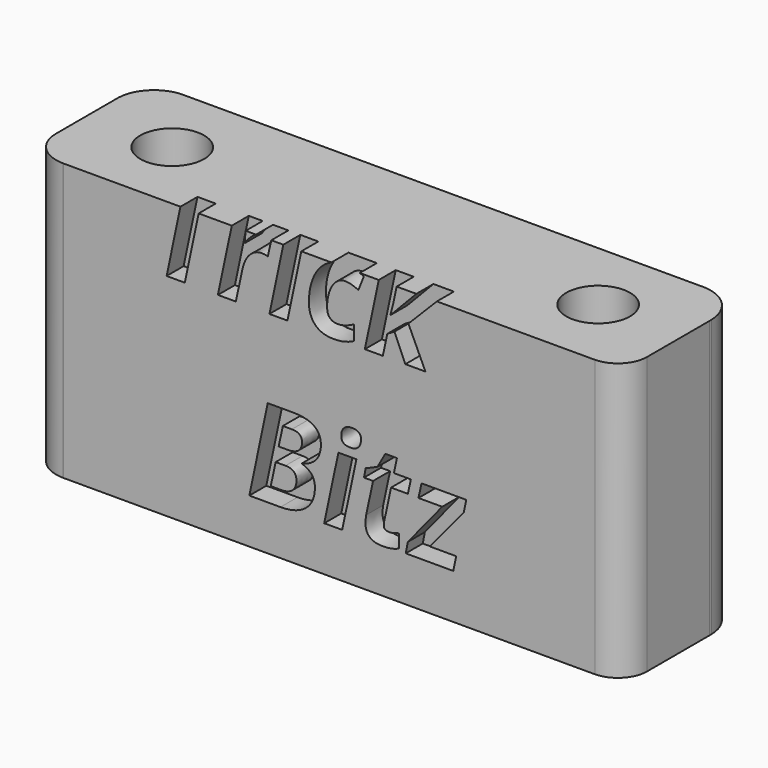
from build123d import *

# Parameters (mm, degrees)
F1_DEPTH     = 13
F2_R         = 1.375
F3_DEPTH     = 10
F4_R         = 1.5
F5_DEPTH     = 10
F6_DEPTH     = 2
F7_TEXT_SIZE = 5.7462564049
F8_DEPTH     = 1
F9_DEPTH     = 2


# Not quite as in the source:
# - Text() gives the source's letters only with a copy of the font that has no kerning and outlines rounded to 1/6400 em; it was checked with that copy


with BuildPart() as f1:
    # F0 (on Top) → F1 (new body)
    with BuildSketch(Plane.XY):
        with BuildLine():
            ThreePointArc((-28, 1.6615508357), (-27.5071954744, 0.4933001093), (-26.3391539245, 0))
            Line((-26.3391539245, 0), (-26.2933354825, 0))
            Line((-26.2933354825, 0), (-1.3435167493, 0))
            ThreePointArc((-1.3435167493, 0), (-0.3933494407, 0.4100272729), (0, 1.3672192581))
            Line((0, 1.3672192581), (0, 5.037621595))
            Line((0, 5.037621595), (0, 5.1521943092))
            ThreePointArc((0, 5.1521943092), (-0.5268150374, 6.4133231242), (-1.7612340162, 7))
            Line((-1.7612340162, 7), (-26.2933354825, 7))
            ThreePointArc((-26.2933354825, 7), (-27.4858583006, 6.507821672), (-28, 5.3246021271))
            Line((-28, 5.3246021271), (-28, 1.6615508357))
        make_face()
        with BuildLine():
            Line((-26.2933354825, 0), (-26.3391539245, 0))
            ThreePointArc((-26.3391539245, 0), (-26.3162447035, -0.0001558454), (-26.2933354825, 0))
        make_face()
        with BuildLine():
            Line((0, 5.1521943092), (0, 5.037621595))
            ThreePointArc((0, 5.037621595), (0.0008588817, 5.0949079521), (0, 5.1521943092))
        make_face()
    extrude(amount=F1_DEPTH)

    # F2 (on face) → F3 (cut)
    with BuildSketch(Plane(origin=(0, 0, 0), x_dir=(1, 0, 0), z_dir=(0, 0, -1))):
        with Locations((-20, -3.5)):
            Circle(F2_R)
        with Locations((-8, -3.5)):
            Circle(F2_R)
    extrude(amount=-F3_DEPTH, mode=Mode.SUBTRACT)

    # F4 (on face) → F5 (cut)
    with BuildSketch(Plane.XY.offset(13)):
        with Locations((-24, 3.5)):
            Circle(F4_R)
        with Locations((-4, 3.5)):
            Circle(F4_R)
    extrude(amount=-F5_DEPTH, mode=Mode.SUBTRACT)

    # F6 (add): a face of the model
    f6_faces = [f1.faces().sort_by_distance(p)[0] for p in [
        (-13.9950424729, 3.4936350813, 0),
    ]]
    extrude(f6_faces, amount=F6_DEPTH)

    # F7 (on face) → F8 (cut)
    with BuildSketch(Plane.XZ):
        with Locations((-22.2090510651, 7.9248473048)):
            Text('Trick', F7_TEXT_SIZE, font='Open Sans', font_style=FontStyle.BOLDITALIC, text_align=(TextAlign.LEFT, TextAlign.BOTTOM))
        with Locations((-17.729664627, 0.1099385942)):
            Text('Bitz', F7_TEXT_SIZE, font='Open Sans', font_style=FontStyle.BOLDITALIC, text_align=(TextAlign.LEFT, TextAlign.BOTTOM))
    extrude(amount=-F8_DEPTH, mode=Mode.SUBTRACT)

    # F9 (cut): a face of the model
    f9_faces = [f1.faces().sort_by_distance(p)[0] for p in [
        (-13.9949800913, 3.4935549902, 13),
    ]]
    extrude(f9_faces, amount=-F9_DEPTH, mode=Mode.SUBTRACT)


solid = f1.part
